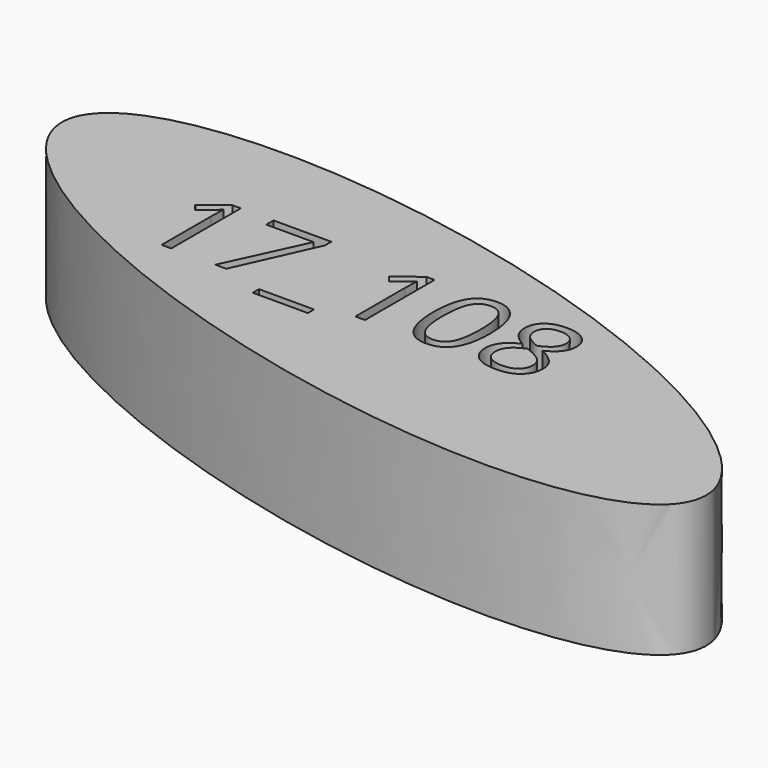
from build123d import *

# Parameters (mm, degrees)
F1_DEPTH     = 25.4
F2_TEXT_SIZE = 23.3390213301
F3_DEPTH     = 25.4


# Not quite as in the source:
# - Text() gives the source's letters only with a copy of the font that has no kerning and outlines rounded to 1/6400 em; it was checked with that copy


with BuildPart() as f1:
    # F0 (on Top) → F1 (new body)
    with BuildSketch(Plane.XY):
        with BuildLine():
            add(Edge.make_bspline(
                [(75.2026066184, -18.9963579178), (85.3715953563, 21.2605409609), (-32.5168089403, 29.6266283982), (-150.4052132368, 37.9927158356), (-42.6857976781, -10.6302704804), (65.0336178806, -59.2532567965), (75.2026066184, -18.9963579178)],
                knots=[0, 0, 0, 2.0943951024, 2.0943951024, 4.1887902048, 4.1887902048, 6.2831853072, 6.2831853072, 6.2831853072], degree=2, weights=[1, 0.5, 1, 0.5, 1, 0.5, 1]))
        make_face()
    extrude(amount=F1_DEPTH)

    # F2 (on face) → F3 (cut)
    with BuildSketch(Plane.XY.offset(25.4)):
        with Locations((-45.2257683501, -4.6380688436)):
            Text('17_108', F2_TEXT_SIZE, font='Open Sans', text_align=(TextAlign.LEFT, TextAlign.BOTTOM))
    extrude(amount=-F3_DEPTH, mode=Mode.SUBTRACT)


solid = f1.part
